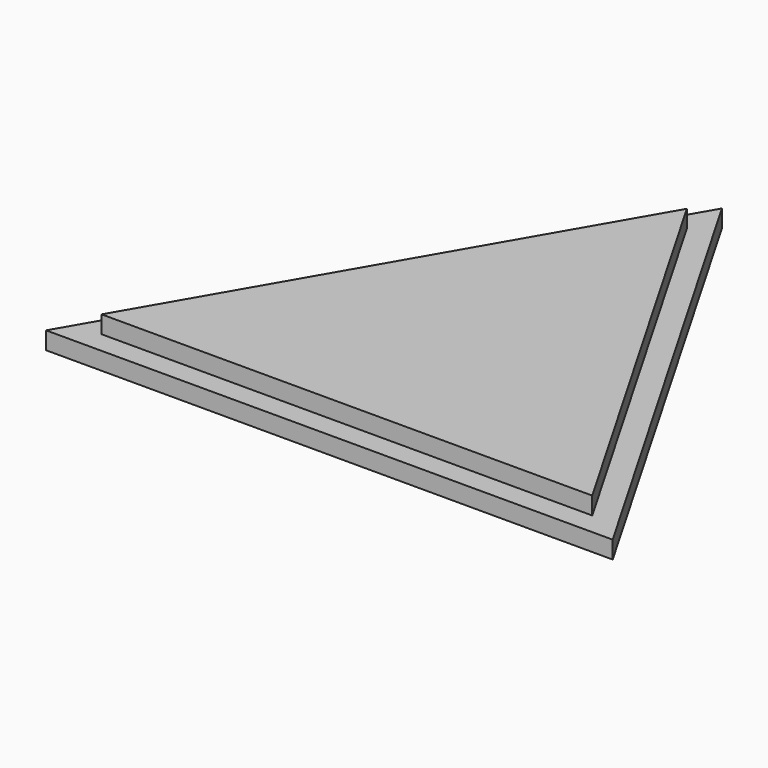
from build123d import *

# Parameters (mm, degrees)
F1_DEPTH = 4
F2_DEPTH = 2
F3_START = 2
F3_DEPTH = 2
F4_SIZE  = 1.99999
F5_R     = 2
F6_DEPTH = 3.75
F7_DEPTH = 3.5
F8_DEPTH = 3.25
F9_DEPTH = 3


# Not quite as in the source:
# - a fillet or chamfer is up to 0.001 mm smaller than in the source, because OpenCascade refuses the exact size


with BuildPart() as f1:
    # F0 (on Top) → F1 (new body)
    with BuildSketch(Plane.XY):
        Polygon((32.7846783229, 14.824549064), (4.8026783229, 63.2907947614), (-23.1793216771, 14.824549064), align=None)
        Polygon((-19.715220062, 16.824549064), (4.8026783229, 59.2907947614), (29.3205767077, 16.824549064), align=None, mode=Mode.SUBTRACT)
    extrude(amount=F1_DEPTH)

    # F0 (on Top) → F2 (join)
    with BuildSketch(Plane.XY):
        Polygon((37.1148053418, 12.324549064), (4.8026783229, 68.2907947614), (-27.509448696, 12.324549064), align=None)
        Polygon((-23.1793216771, 14.824549064), (4.8026783229, 63.2907947614), (32.7846783229, 14.824549064), align=None, mode=Mode.SUBTRACT)
    extrude(amount=F2_DEPTH)

    # F0 (on Top) → F3 (join)
    with BuildSketch(Plane.XY.offset(F3_START)):
        Polygon((29.3205767077, 16.824549064), (4.8026783229, 59.2907947614), (-19.715220062, 16.824549064), align=None)
    extrude(amount=F3_DEPTH)

    # F4 (size 2 in the source; OpenCascade refuses exactly that, so slightly less here)
    f4_edges = [f1.edges().sort_by_distance(p)[0] for p in [
        (4.802678, 16.824549, 0),
        (-7.456271, 38.057672, 0),
        (17.061628, 38.057672, 0),
    ]]
    chamfer(f4_edges, length=F4_SIZE)

    # F5 (on face) → F6 (cut)
    with BuildSketch(Plane.XY):
        with BuildLine():
            Line((15.8012454512, 40.2407176847), (14.8071694273, 41.9625078646))
            ThreePointArc((14.8071694273, 41.9625078646), (12.0675004242, 39.2368445398), (15.801257126, 40.2338840067))
            ThreePointArc((15.801257126, 40.2338840067), (15.8012542073, 40.2373008507), (15.8012454512, 40.2407176847))
        make_face()
        with Locations((-10.6723830104, 23.3052875847)):
            Circle(F5_R)
    extrude(amount=F6_DEPTH, mode=Mode.SUBTRACT)

    # F5 (on face) → F7 (cut)
    with BuildSketch(Plane.XY):
        with BuildLine():
            Line((3.6860700174, 34.755180139), (9.4204377363, 37.8238173116))
            ThreePointArc((9.4204377363, 37.8238173116), (9.2694965624, 38.1212680469), (9.1387235678, 38.4281207834))
            Line((9.1387235678, 38.4281207834), (0.9941436583, 35.2838113904))
            Line((0.9941436583, 35.2838113904), (-2.8154677711, 33.8130667806))
            Line((-2.8154677711, 33.8130667806), (1.0452440474, 33.3419926465))
            Line((1.0452440474, 33.3419926465), (3.6860700174, 34.755180139))
        make_face()
        with BuildLine():
            Line((17.0693753854, 23.8813530259), (14.9441122519, 35.3662478082))
            ThreePointArc((14.9441122519, 35.3662478082), (14.2087911946, 35.2505200844), (13.4644377158, 35.2452416378))
            Line((13.4644377158, 35.2452416378), (12.8494622186, 26.1368211359))
            Line((12.8494622186, 26.1368211359), (15.8132929355, 24.552706629))
            Line((15.8132929355, 24.552706629), (17.0693753854, 23.8813530259))
        make_face()
        with BuildLine():
            Line((-13.4587365793, 16.824549064), (-6.1025659626, 16.824549064))
            Line((-6.1025659626, 16.824549064), (-3.819498702, 19.0105444595))
            Line((-3.819498702, 19.0105444595), (-1.2189327972, 21.5005390346))
            Line((-1.2189327972, 21.5005390346), (-7.725601985, 22.742720621))
            ThreePointArc((-7.725601985, 22.742720621), (-9.2656609828, 20.6555454959), (-11.8573356204, 20.5492238495))
            Line((-11.8573356204, 20.5492238495), (-13.4587365793, 16.824549064))
        make_face()
        with BuildLine():
            ThreePointArc((9.6781818277, 43.0623553402), (10.154568974, 43.6546537332), (10.7152328484, 44.1678964823))
            Line((10.7152328484, 44.1678964823), (5.5434275419, 50.7608279586))
            Line((5.5434275419, 50.7608279586), (5.1609951292, 49.6271412781))
            Line((5.1609951292, 49.6271412781), (4.2115291581, 46.8125343323))
            Line((4.2115291581, 46.8125343323), (9.6781818277, 43.0623553402))
        make_face()
    extrude(amount=F7_DEPTH, mode=Mode.SUBTRACT)

    # F5 (on face) → F8 (cut)
    with BuildSketch(Plane.XY):
        with BuildLine():
            Line((19.8564007878, 24.4885329157), (15.5959561349, 35.5670804467))
            ThreePointArc((15.5959561349, 35.5670804467), (15.2734627879, 35.4555359146), (14.9441122519, 35.3662478082))
            Line((14.9441122519, 35.3662478082), (17.0693753854, 23.8813530259))
            Line((17.0693753854, 23.8813530259), (15.8132929355, 24.552706629))
            Line((15.8132929355, 24.552706629), (17.4690298736, 20.0315453112))
            Line((17.4690298736, 20.0315453112), (19.8564007878, 24.4885329157))
        make_face()
        Polygon((-6.1025659626, 16.824549064), (1.2875116271, 16.824549064), (1.7734020948, 17.1169545501), (-3.819498702, 19.0105444595), align=None)
        with BuildLine():
            Line((5.785849411, 33.66388008), (9.9342960343, 37.064244924))
            ThreePointArc((9.9342960343, 37.064244924), (9.6599157648, 37.4322252607), (9.4204377363, 37.8238173116))
            Line((9.4204377363, 37.8238173116), (3.6860700174, 34.755180139))
            Line((3.6860700174, 34.755180139), (5.785849411, 33.66388008))
        make_face()
        with BuildLine():
            ThreePointArc((11.5326481984, 44.6896009562), (11.8941525727, 44.8558913869), (12.2677356256, 44.9929082563))
            Line((12.2677356256, 44.9929082563), (11.2701070238, 48.0888796571))
            Line((11.2701070238, 48.0888796571), (7.7075759005, 54.2593645662))
            Line((7.7075759005, 54.2593645662), (6.1958078295, 55.1715530455))
            Line((6.1958078295, 55.1715530455), (7.7216781624, 52.1746300315))
            Line((7.7216781624, 52.1746300315), (11.5326481984, 44.6896009562))
        make_face()
        with BuildLine():
            ThreePointArc((-12.7082549566, 21.1018299793), (-12.079105038, 25.9550296735), (-7.7066088949, 23.7571547066))
            Line((-7.7066088949, 23.7571547066), (-6.6805827438, 23.5612770993))
            ThreePointArc((-6.6805827438, 23.5612770993), (-12.5480123805, 26.8382770364), (-13.1208381636, 20.1422088056))
            Line((-13.1208381636, 20.1422088056), (-12.7082549566, 21.1018299793))
        make_face()
    extrude(amount=F8_DEPTH, mode=Mode.SUBTRACT)

    # F5 (on face) → F9 (cut)
    with BuildSketch(Plane.XY):
        with BuildLine():
            ThreePointArc((9.1387235678, 38.4281207834), (8.9697402045, 38.9468547775), (8.8582790135, 39.4809116441))
            Line((8.8582790135, 39.4809116441), (1.4540485572, 38.196541369))
            Line((1.4540485572, 38.196541369), (0.9941436583, 35.2838113904))
            Line((0.9941436583, 35.2838113904), (9.1387235678, 38.4281207834))
        make_face()
        with BuildLine():
            ThreePointArc((10.7152328484, 44.1678964823), (11.1112630591, 44.4486119837), (11.5326481984, 44.6896009562))
            Line((11.5326481984, 44.6896009562), (7.7216781624, 52.1746300315))
            Line((7.7216781624, 52.1746300315), (3.6355266348, 51.2855537236))
            Line((3.6355266348, 51.2855537236), (5.1609951292, 49.6271412781))
            Line((5.1609951292, 49.6271412781), (5.5434275419, 50.7608279586))
            Line((5.5434275419, 50.7608279586), (10.7152328484, 44.1678964823))
        make_face()
    extrude(amount=F9_DEPTH, mode=Mode.SUBTRACT)


solid = f1.part
